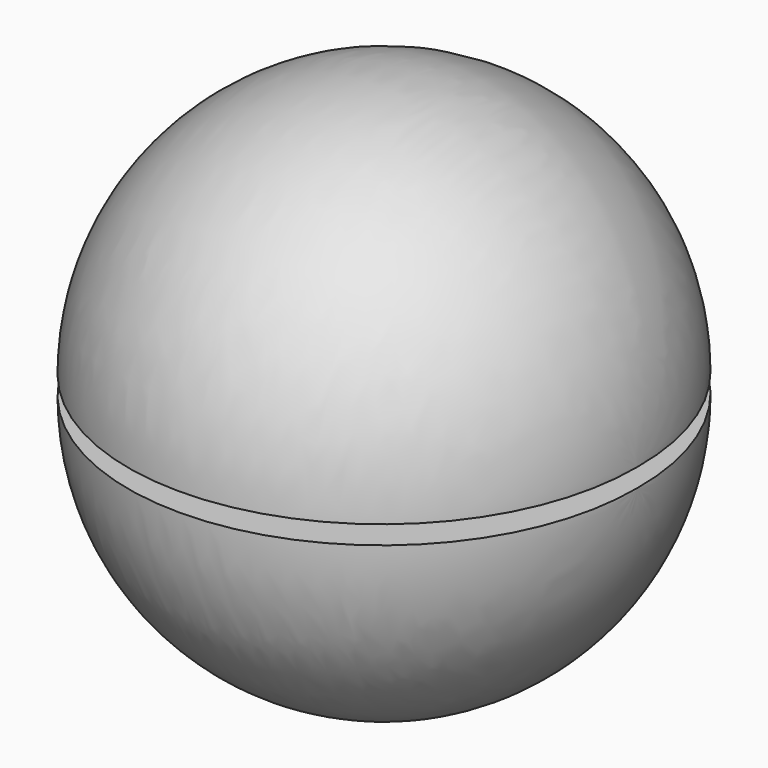
from build123d import *

# Parameters (mm, degrees)
F1_ANGLE = 180
F2_W     = 27.4360350213
F2_H     = 1.27
F8_DEPTH = 38.1


# Not quite as in the source:
# - the program builds the solid bodies; features that only make, move or delete a surface that nothing else refers to are left out


with BuildPart() as f1:
    # F0 (on Top) → F1 (revolve)
    with BuildSketch(Plane.XY):
        with BuildLine():
            Line((32.5160350213, 0), (-36.8259649787, 0))
            ThreePointArc((-36.8259649787, 0), (-2.1549649787, -35.0073002846), (32.5160350213, 0))
        make_face()
    revolve(axis=Axis((-2.1549649787, 0, 0), (-1, 0, 0)), revolution_arc=F1_ANGLE)

    # F2 (on Front) → F3 (revolve)
    with BuildSketch(Plane.XZ):
        with Locations((13.7180175106, -0.635)):
            Rectangle(F2_W, F2_H)
    revolve(axis=Axis((0, 0, -0.635), (0, 0, -1)))

    # F4: F1 across face


with BuildPart() as f1_1:
    add(f1.part)
    add(f1.part.mirror(Plane(origin=(0, 0, -1.27), x_dir=(1, 0, 0), z_dir=(0, 0, -1))))

    # F7 (on Right) → F8 (join)
    with BuildSketch(Plane.YZ):
        with BuildLine():
            ThreePointArc((-0.7505157715, 4.4294735411), (-4.7934462503, -8.0205740429), (7.1645930807, -2.6957015507))
            ThreePointArc((7.1645930807, -2.6957015507), (4.7934462503, 2.6291709415), (-0.7505157715, 4.4294735411))
        make_face()
    extrude(amount=-F8_DEPTH)


solid = f1_1.part
